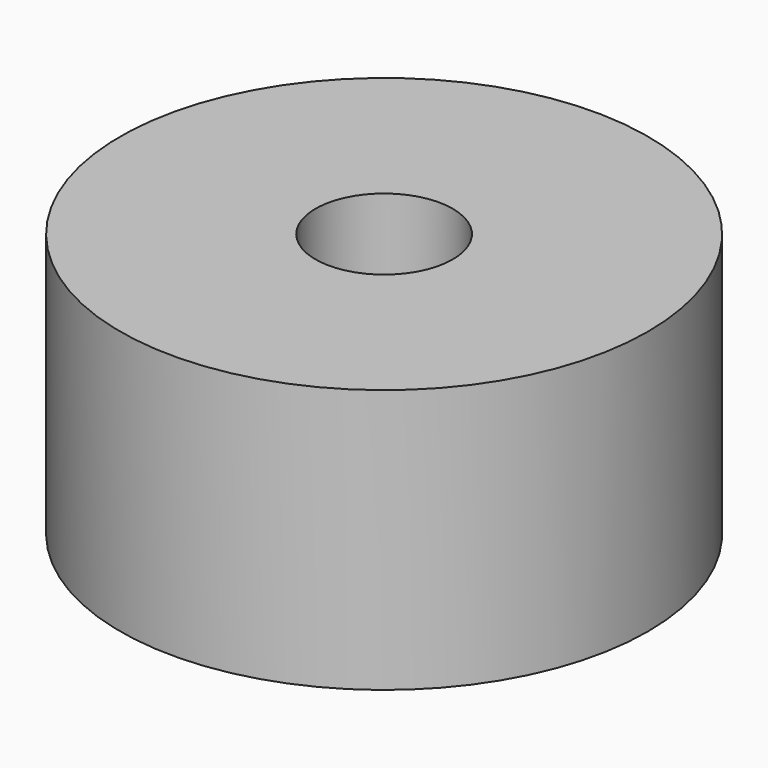
from build123d import *

# Parameters (mm, degrees)
F0_R     = 12.7
F0_R_2   = 3.302
F1_DEPTH = 12.7


# Not quite as in the source:
# - the program builds the solid bodies; features that only make, move or delete a surface that nothing else refers to are left out


with BuildPart() as f1:
    # F0 (on Top) → F1 (new body)
    with BuildSketch(Plane.XY):
        Circle(F0_R)
        Circle(F0_R_2, mode=Mode.SUBTRACT)
    extrude(amount=F1_DEPTH)


solid = f1.part
